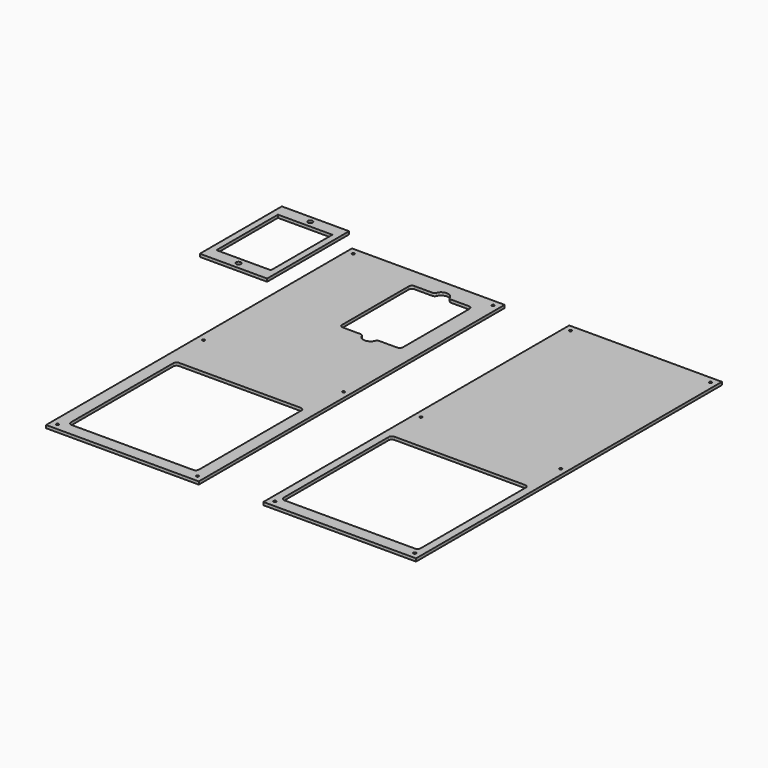
from build123d import *

# Parameters (mm, degrees)
F0_W         = 238.4
F0_H         = 597
F0_W_2       = 200
F0_H_2       = 210
F1_DEPTH     = 4.5
F3_D         = 4
F4_W         = 238.4
F4_H         = 597
F4_W_2       = 214
F4_H_2       = 215
F5_DEPTH     = 4.5
F7_D         = 4
F8_R         = 5
F9_R         = 5
F10_R        = 5
F11_W        = 105
F11_H        = 160
F12_DEPTH    = 4.5
F13_W        = 85
F13_H        = 120
F13_R        = 3.75
F14_DEPTH    = 25
F15_W        = 22
F15_H        = 160
F16_DEPTH    = 25
F17_T1_DEPTH = 4.5
F18_R        = 5


# Not quite as in the source:
# - a fillet or chamfer that OpenCascade refuses, or shapes differently, is made with other operations: its cross-section is extruded or revolved along the edge and cut away or added


with BuildPart() as f1:
    # F0 (on Top) → F1 (new body)
    with BuildSketch(Plane.XY):
        with Locations((-86.8, 100.3010249138)):
            Rectangle(F0_W, F0_H)
        with Locations((-86.8, -73.7989750862)):
            Rectangle(F0_W_2, F0_H_2, mode=Mode.SUBTRACT)
        with BuildLine():
            ThreePointArc((-52.6800657034, 368.8010249138), (-49.4800657034, 372.0010249138), (-46.2800657034, 368.8010249138))
            Line((-46.2800657034, 368.8010249138), (5.6, 368.8010249138))
            Line((5.6, 368.8010249138), (5.6, 228.8010249138))
            Line((5.6, 228.8010249138), (-89.4, 228.8010249138))
            Line((-89.4, 228.8010249138), (-89.4, 368.8010249138))
            Line((-89.4, 368.8010249138), (-52.6800657034, 368.8010249138))
        make_face(mode=Mode.SUBTRACT)
    extrude(amount=F1_DEPTH)

    # F3 (through all)
    with Locations(Plane.XY.offset(4.5)):
        with Locations((-196, 388.8010249138), (22.4, 388.8010249138), (22.4, 96.8010249138), (-196, 96.8010249138), (-196, -188.1989750862), (22.4, -188.1989750862)):
            Hole(F3_D / 2)

    # F9
    f9_edges = [f1.edges().sort_by_distance(p)[0] for p in [
        (13.2, 31.201025, 2.25),
        (-186.8, 31.201025, 2.25),
        (13.2, -178.798975, 2.25),
        (-186.8, -178.798975, 2.25),
    ]]
    fillet(f9_edges, radius=F9_R)

    # F10
    f10_edges = [f1.edges().sort_by_distance(p)[0] for p in [
        (-89.4, 368.801025, 2.25),
        (5.6, 368.801025, 2.25),
        (5.6, 228.801025, 2.25),
        (-89.4, 228.801025, 2.25),
    ]]
    fillet(f10_edges, radius=F10_R)

    # F15 (on face) → F16 (cut)
    with BuildSketch(Plane.XY.offset(4.5)):
        with Locations((-41.9, 298.8010249138)):
            Rectangle(F15_W, F15_H)
    extrude(amount=-F16_DEPTH, mode=Mode.SUBTRACT)

    # F17: fillet of radius 11 on 4 edges, made by hand

    # F17_s2 → F17_t1 (join)
    with BuildSketch(Plane.XY):
        with BuildLine():
            ThreePointArc((-30.9, 368.8010249138), (-34.438252663, 375.9250633184), (-41.8544511501, 378.8010249138))
            Line((-41.8544511501, 378.8010249138), (-30.9, 378.8010249138))
            Line((-30.9, 378.8010249138), (-30.9, 368.8010249138))
        make_face()
        with BuildLine():
            ThreePointArc((-41.9455488499, 378.8010249138), (-49.361747337, 375.9250633184), (-52.9, 368.8010249138))
            Line((-52.9, 368.8010249138), (-52.9, 378.8010249138))
            Line((-52.9, 378.8010249138), (-41.9455488499, 378.8010249138))
        make_face()
        with BuildLine():
            ThreePointArc((-52.9, 228.8010249138), (-49.361747337, 221.6769865092), (-41.9455488499, 218.8010249138))
            Line((-41.9455488499, 218.8010249138), (-52.9, 218.8010249138))
            Line((-52.9, 218.8010249138), (-52.9, 228.8010249138))
        make_face()
        with BuildLine():
            ThreePointArc((-41.8544511501, 218.8010249138), (-34.438252663, 221.6769865092), (-30.9, 228.8010249138))
            Line((-30.9, 228.8010249138), (-30.9, 218.8010249138))
            Line((-30.9, 218.8010249138), (-41.8544511501, 218.8010249138))
        make_face()
    extrude(amount=F17_T1_DEPTH)

    # F18
    f18_edges = [f1.edges().sort_by_distance(p)[0] for p in [
        (-52.9, 368.801025, 2.25),
        (-30.9, 368.801025, 2.25),
        (-30.9, 228.801025, 2.25),
        (-52.9, 228.801025, 2.25),
    ]]
    fillet(f18_edges, radius=F18_R)


with BuildPart() as f5:
    # F4 (on Top) → F5 (new body)
    with BuildSketch(Plane.XY):
        with Locations((247.0295269012, 107.0325807333)):
            Rectangle(F4_W, F4_H)
        with Locations((247.0295269012, -64.5674192667)):
            Rectangle(F4_W_2, F4_H_2, mode=Mode.SUBTRACT)
    extrude(amount=F5_DEPTH)

    # F7 (through all)
    with Locations(Plane.XY.offset(4.5)):
        with Locations((137.8295269012, 395.5325807333), (356.2295269012, 395.5325807333), (356.2295269012, 103.5325807333), (137.8295269012, 103.5325807333), (137.8295269012, -181.4674192667), (356.2295269012, -181.4674192667)):
            Hole(F7_D / 2)

    # F8
    f8_edges = [f5.edges().sort_by_distance(p)[0] for p in [
        (354.029527, 42.932581, 2.25),
        (140.029527, 42.932581, 2.25),
        (354.029527, -172.067419, 2.25),
        (140.029527, -172.067419, 2.25),
    ]]
    fillet(f8_edges, radius=F8_R)


with BuildPart() as f12:
    # F11 (on Top) → F12 (new body)
    with BuildSketch(Plane.XY):
        with Locations((-289.6022295952, 352.065103054)):
            Rectangle(F11_W, F11_H)
    extrude(amount=F12_DEPTH)

    # F13 (on face) → F14 (cut)
    with BuildSketch(Plane.XY.offset(4.5)):
        with Locations((-289.6849620342, 352.065103054)):
            Rectangle(F13_W, F13_H)
        with Locations((-289.6022295952, 422.065103054)):
            Circle(F13_R)
        with Locations((-289.6022295952, 282.065103054)):
            Circle(F13_R)
    extrude(amount=-F14_DEPTH, mode=Mode.SUBTRACT)


solid = Compound([f1.part, f5.part, f12.part])
